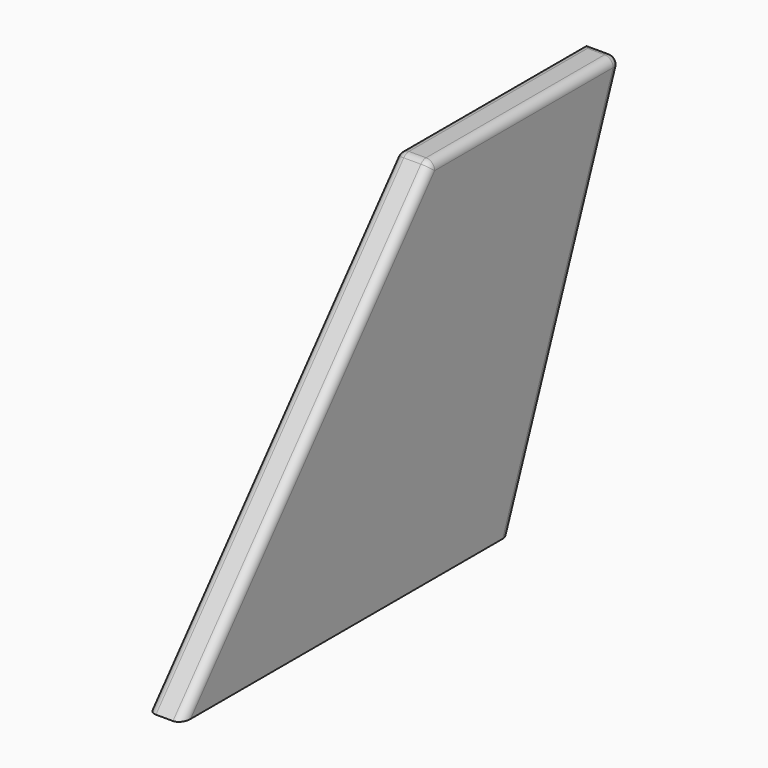
from build123d import *

# Parameters (mm, degrees)
F2_DEPTH     = 100
F3_R         = 50
F4_T1_DEPTH  = 1304.0811873082
F4_T3_DEPTH  = 1501.8872234652
F4_T5_DEPTH  = 332.0150903927
F4_T7_DEPTH  = 100
F4_T12_DEPTH = 50
F4_T18_DEPTH = 50
F4_T24_DEPTH = 50


# Not quite as in the source:
# - a fillet or chamfer that OpenCascade refuses, or shapes differently, is made with other operations: its cross-section is extruded or revolved along the edge and cut away or added


with BuildPart() as f2:
    # F0 (on Right) → F2 (new body, symmetric)
    with BuildSketch(Plane.YZ):
        Polygon((507.0400096967, 2146.646806384), (-1318.7368903443, 0), (1081.2631096557, 0), (1907.0400096967, 2146.646806384), align=None)
    extrude(amount=F2_DEPTH, both=True)

    # F3
    f3_edges = [f2.edges().sort_by_distance(p)[0] for p in [
        (-100, -405.84844, 1073.323403),
        (100, -405.84844, 1073.323403),
        (100, 1494.15156, 1073.323403),
    ]]
    fillet(f3_edges, radius=F3_R)

    # F4: fillet of radius 50 on 4 edges, made by hand

    # F4_s2 → F4_t1 (cut)
    with BuildSketch(Plane.XZ.offset(-1834.2339735396)):
        with BuildLine():
            ThreePointArc((50, 2146.646806384), (85.3553390593, 2132.0021454433), (100, 2096.646806384))
            Line((100, 2096.646806384), (100, 2146.646806384))
            Line((100, 2146.646806384), (50, 2146.646806384))
        make_face()
    extrude(amount=F4_T1_DEPTH, mode=Mode.SUBTRACT)

    # F4_s4 → F4_t3 (cut)
    with BuildSketch(Plane.XZ.offset(-2032.0400096967)):
        with BuildLine():
            ThreePointArc((-50, 2146.646806384), (-85.3553390593, 2132.0021454433), (-100, 2096.646806384))
            Line((-100, 2096.646806384), (-100, 2146.646806384))
            Line((-100, 2146.646806384), (-50, 2146.646806384))
        make_face()
    extrude(amount=F4_T3_DEPTH, mode=Mode.SUBTRACT)

    # F4_s6 → F4_t5 (cut)
    with BuildSketch(Plane.YZ.offset(-282.0150903927)):
        with BuildLine():
            ThreePointArc((1834.2339735396, 2146.646806384), (1875.4503755357, 2124.9524278487), (1880.900208461, 2078.695134644))
            Line((1880.900208461, 2078.695134644), (1907.0400096967, 2146.646806384))
            Line((1907.0400096967, 2146.646806384), (1834.2339735396, 2146.646806384))
        make_face()
    extrude(amount=F4_T5_DEPTH, mode=Mode.SUBTRACT)

    # F4_s8 → F4_t7 (cut)
    with BuildSketch(Plane.YZ.offset(-50)):
        with BuildLine():
            ThreePointArc((530.1527862314, 2146.646806384), (509.1730515679, 2142.0323848583), (492.0656904737, 2129.0408357219))
            Line((492.0656904737, 2129.0408357219), (507.0400096967, 2146.646806384))
            Line((507.0400096967, 2146.646806384), (530.1527862314, 2146.646806384))
        make_face()
    extrude(amount=F4_T7_DEPTH, mode=Mode.SUBTRACT)


with BuildPart() as f4_tool10:
    # F4_s11 → F4_t12 (new body)
    with BuildSketch(Plane.YZ.offset(-50)):
        Polygon((530.1527862314, 2096.646806384), (492.0656904737, 2129.0408357219), (507.0400096967, 2146.646806384), (530.1527862314, 2146.646806384), align=None)
    extrude(amount=-F4_T12_DEPTH)

    # F4_s13 → F4_t14 (revolve, cut)
    with BuildSketch(Plane(origin=(-50, 530.1527862314, 2096.646806384), x_dir=(0, 0.4195946933, -0.9077115695), z_dir=(0, 0.9077115695, 0.4195946933))):
        with BuildLine():
            ThreePointArc((0, -50), (50, 0), (0, 50))
            Line((0, 50), (0, -50))
        make_face()
    revolve(axis=Axis((-50, 530.1527862314, 2096.646806384), (-1, 0, 0)), mode=Mode.SUBTRACT)


with BuildPart() as f2_1:
    add(f2.part)

    # F4_t9: cut F4_tool10
    add(f4_tool10.part, mode=Mode.SUBTRACT)


with BuildPart() as f4_tool16:
    # F4_s17 → F4_t18 (new body)
    with BuildSketch(Plane.YZ.offset(50)):
        Polygon((530.1527862314, 2096.646806384), (530.1527862314, 2146.646806384), (507.0400096967, 2146.646806384), (492.0656904737, 2129.0408357219), align=None)
    extrude(amount=F4_T18_DEPTH)

    # F4_s19 → F4_t20 (revolve, cut)
    with BuildSketch(Plane(origin=(50, 530.1527862314, 2096.646806384), x_dir=(0, 0.4195946933, -0.9077115695), z_dir=(0, -0.9077115695, -0.4195946933))):
        with BuildLine():
            ThreePointArc((0, -50), (50, 0), (0, 50))
            Line((0, 50), (0, -50))
        make_face()
    revolve(axis=Axis((50, 530.1527862314, 2096.646806384), (1, 0, 0)), mode=Mode.SUBTRACT)


with BuildPart() as f2_2:
    add(f2_1.part)

    # F4_t15: cut F4_tool16
    add(f4_tool16.part, mode=Mode.SUBTRACT)


with BuildPart() as f4_tool22:
    # F4_s23 → F4_t24 (new body)
    with BuildSketch(Plane.YZ.offset(50)):
        Polygon((1834.2339735396, 2096.646806384), (1834.2339735396, 2146.646806384), (1907.0400096967, 2146.646806384), (1880.900208461, 2078.695134644), align=None)
    extrude(amount=F4_T24_DEPTH)

    # F4_s25 → F4_t26 (revolve, cut)
    with BuildSketch(Plane(origin=(50, 1834.2339735396, 2096.646806384), x_dir=(0, -0.8243280399, -0.5661124293), z_dir=(0, -0.5661124293, 0.8243280399))):
        with BuildLine():
            ThreePointArc((0, -50), (50, 0), (0, 50))
            Line((0, 50), (0, -50))
        make_face()
    revolve(axis=Axis((50, 1834.2339735396, 2096.646806384), (1, 0, 0)), mode=Mode.SUBTRACT)


with BuildPart() as f2_3:
    add(f2_2.part)

    # F4_t21: cut F4_tool22
    add(f4_tool22.part, mode=Mode.SUBTRACT)


solid = f2_3.part
